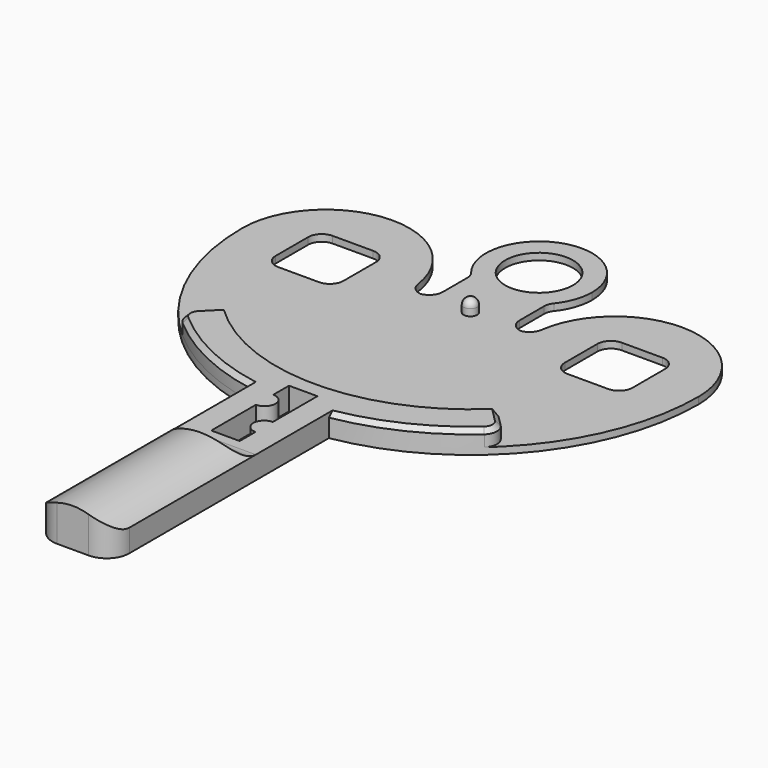
from build123d import *

# Parameters (mm, degrees)
F1_DEPTH     = 5
F3_DEPTH     = 5.001
F5_DEPTH     = 35
F6_T4_DEPTH  = 17.0072864353
F6_S5_R      = 12
F6_T6_DEPTH  = 11
F6_T7_DEPTH  = 30
F7_R         = 7.5
F8_DEPTH     = 5
F9_R         = 45.5
F10_DEPTH    = 3.5
F12_DEPTH    = 1.5
F14_DEPTH    = 3.5
F18_W        = 15
F18_H        = 15
F19_DEPTH    = 1.5010001
F20_DEPTH    = 5.0010001
F21_R        = 1.5
F22_DEPTH    = 3
F23_T1_DEPTH = 1.5
F23_T3_DEPTH = 11.4776669635
F24_R        = 1.5
F25_SIZE     = 1


# Not quite as in the source:
# - a fillet or chamfer that OpenCascade refuses, or shapes differently, is made with other operations: its cross-section is extruded or revolved along the edge and cut away or added
# - a feature names something its author has since deleted; it is built from what else it names


with BuildPart() as f1:
    # F0 (on Top) → F1 (new body)
    with BuildSketch(Plane.XY):
        Polygon((8.5036432176, -40), (-8.5036432176, -40), (-8.5036432176, -110), (0, -110), (8.5036432176, -110), align=None)
    extrude(amount=F1_DEPTH)

    # F2 (on face) → F3 (cut, through all)
    with BuildSketch(Plane.XY.offset(5)):
        with BuildLine():
            Line((-3.15, -67.75), (3.15, -67.75))
            Line((3.15, -67.75), (3.15, -63.4))
            ThreePointArc((3.15, -63.4), (0.75, -61), (3.15, -58.6))
            Line((3.15, -58.6), (3.15, -46.25))
            Line((3.15, -46.25), (-3.15, -46.25))
            Line((-3.15, -46.25), (-3.15, -50.6))
            ThreePointArc((-3.15, -50.6), (-0.75, -53), (-3.15, -55.4))
            Line((-3.15, -55.4), (-3.15, -67.75))
        make_face()
    extrude(amount=-F3_DEPTH, mode=Mode.SUBTRACT)

    # F4 (on face) → F5 (join)
    with BuildSketch(Plane.XZ.offset(110)):
        with BuildLine():
            ThreePointArc((8.5036432176, 5), (0, 8.5331202898), (-8.5036432176, 5))
            Line((-8.5036432176, 5), (8.5036432176, 5))
        make_face()
    extrude(amount=-F5_DEPTH)

    # F6: fillet of radius 5 on 3 edges, made by hand


with BuildPart() as f6_tool2:
    # F6_s3 → F6_t4 (new body)
    with BuildSketch(Plane.YZ.offset(-8.5036432176)):
        with BuildLine():
            ThreePointArc((-70, 5), (-73.5355339059, 6.4644660941), (-75, 10))
            Line((-75, 10), (-75, 5))
            Line((-75, 5), (-70, 5))
        make_face()
    extrude(amount=F6_T4_DEPTH)

    # F6_s5 → F6_t6 (intersect, symmetric)
    with BuildSketch(Plane.XZ.offset(72.5)):
        with Locations((0, -3.4668797102)):
            Circle(F6_S5_R)
    extrude(amount=F6_T6_DEPTH, both=True, mode=Mode.INTERSECT)


with BuildPart() as f1_1:
    add(f1.part)

    # F6_t1: union F6_tool2
    add(f6_tool2.part)

    # F6_s8 → F6_t7 (cut)
    with BuildSketch(Plane.XY.offset(-12.5)):
        with BuildLine():
            ThreePointArc((-8.5036432176, -105), (-7.0391771236, -108.5355339059), (-3.5036432176, -110))
            Line((-3.5036432176, -110), (-8.5036432176, -110))
            Line((-8.5036432176, -110), (-8.5036432176, -105))
        make_face()
        with BuildLine():
            ThreePointArc((8.5036432176, -105), (7.0391771236, -108.5355339059), (3.5036432176, -110))
            Line((3.5036432176, -110), (8.5036432176, -110))
            Line((8.5036432176, -110), (8.5036432176, -105))
        make_face()
    extrude(amount=F6_T7_DEPTH, mode=Mode.SUBTRACT)

    # F7 (on Top) → F8 (join)
    with BuildSketch(Plane.XY):
        with BuildLine():
            Line((-8.5036432176, 0), (-8.5036432176, -40))
            Line((-8.5036432176, -40), (8.5036432176, -40))
            Line((8.5036432176, -40), (8.5036432176, 0))
            Line((8.5036432176, 0), (8.5036432176, 10.8923699759))
            ThreePointArc((8.5036432176, 10.8923699759), (0, 7.2507186355), (-8.5036432176, 10.8923699759))
            Line((-8.5036432176, 10.8923699759), (-8.5036432176, 0))
        make_face()
        with BuildLine():
            ThreePointArc((11.7492813645, 19), (-4.3665727862, 29.9077337098), (-8.5036432176, 10.8923699759))
            ThreePointArc((-8.5036432176, 10.8923699759), (0, 7.2507186355), (8.5036432176, 10.8923699759))
            ThreePointArc((8.5036432176, 10.8923699759), (10.9077337098, 14.6334272138), (11.7492813645, 19))
        make_face()
        with Locations((0, 19)):
            Circle(F7_R, mode=Mode.SUBTRACT)
    extrude(amount=F8_DEPTH)

    # F9 (on face) → F10 (cut)
    with BuildSketch(Plane.XY.offset(5)):
        Circle(F9_R)
    extrude(amount=-F10_DEPTH, mode=Mode.SUBTRACT)

    # F11 (on Top) → F12 (join)
    with BuildSketch(Plane.XY):
        with BuildLine():
            ThreePointArc((-13.5, 0), (-32, 18.5), (-50.5, 0))
            ThreePointArc((-50.5, 0), (0, -50.5), (50.5, 0))
            ThreePointArc((50.5, 0), (32, 18.5), (13.5, 0))
            Line((13.5, 0), (-13.5, 0))
        make_face()
    extrude(amount=F12_DEPTH)

    # F13 (on face) → F14 (join)
    with BuildSketch(Plane.XY.offset(1.5)):
        with BuildLine():
            ThreePointArc((32.173358544, -32.173358544), (0, -45.5), (-32.173358544, -32.173358544))
            Line((-32.173358544, -32.173358544), (-35.7088924499, -35.7088924499))
            ThreePointArc((-35.7088924499, -35.7088924499), (0, -50.5), (35.7088924499, -35.7088924499))
            Line((35.7088924499, -35.7088924499), (32.173358544, -32.173358544))
        make_face()
    extrude(amount=F14_DEPTH)

    # F17: sweep along a path in F17_path
    with BuildLine(Plane(origin=(32.173358544, -32.173358544, 5), x_dir=(0, 1, 0), z_dir=(0, 0, 1))) as f17_path:
        ThreePointArc((0, 0), (-13.326641456, 32.173358544), (0, 64.346717088))
    # F16 (on face) → F17 (sweep)
    with BuildSketch(Plane(origin=(0, 0, 0), x_dir=(0.7071067812, 0.7071067812, 0), z_dir=(0.7071067812, -0.7071067812, 0))):
        Polygon((-43, 5), (-45.5, 5), (-45.5, 2.5), align=None)
    sweep(path=f17_path.line)

    # F18 (on face) → F19 (cut, through all)
    with BuildSketch(Plane.XY.offset(1.5)):
        with Locations((-32, 0)):
            Rectangle(F18_W, F18_H)
        with Locations((32, 0)):
            Rectangle(F18_W, F18_H)
    extrude(amount=-F19_DEPTH, mode=Mode.SUBTRACT)

    # F2 (on face) → F20 (cut, through all)
    with BuildSketch(Plane.XY.offset(5)):
        with BuildLine():
            Line((-3.15, -67.75), (3.15, -67.75))
            Line((3.15, -67.75), (3.15, -63.4))
            ThreePointArc((3.15, -63.4), (0.75, -61), (3.15, -58.6))
            Line((3.15, -58.6), (3.15, -46.25))
            Line((3.15, -46.25), (-3.15, -46.25))
            Line((-3.15, -46.25), (-3.15, -50.6))
            ThreePointArc((-3.15, -50.6), (-0.75, -53), (-3.15, -55.4))
            Line((-3.15, -55.4), (-3.15, -67.75))
        make_face()
    extrude(amount=-F20_DEPTH, mode=Mode.SUBTRACT)

    # F21 (on face) → F22 (join)
    with BuildSketch(Plane.XY.offset(1.5)):
        Circle(F21_R)
    extrude(amount=F22_DEPTH)

    # F23: fillet of radius 3 on 16 edges, made by hand

    # F23_s2 → F23_t1 (join)
    with BuildSketch(Plane.XY):
        with BuildLine():
            ThreePointArc((-10.710331144, 0), (-12.6780946011, 0.7355117627), (-13.6809826122, 2.5813953488))
            ThreePointArc((-13.6809826122, 2.5813953488), (-13.5453011177, 1.2938659758), (-13.5, 0))
            Line((-13.5, 0), (-10.710331144, 0))
        make_face()
        with BuildLine():
            ThreePointArc((13.6809826122, 2.5813953488), (12.6780946011, 0.7355117627), (10.710331144, 0))
            Line((10.710331144, 0), (13.5, 0))
            ThreePointArc((13.5, 0), (13.5453011177, 1.2938659758), (13.6809826122, 2.5813953488))
        make_face()
        with BuildLine():
            ThreePointArc((39.5, -4.5), (38.6213203436, -6.6213203436), (36.5, -7.5))
            Line((36.5, -7.5), (39.5, -7.5))
            Line((39.5, -7.5), (39.5, -4.5))
        make_face()
        with BuildLine():
            ThreePointArc((24.5, -4.5), (25.3786796564, -6.6213203436), (27.5, -7.5))
            Line((27.5, -7.5), (24.5, -7.5))
            Line((24.5, -7.5), (24.5, -4.5))
        make_face()
        with BuildLine():
            ThreePointArc((24.5, 4.5), (25.3786796564, 6.6213203436), (27.5, 7.5))
            Line((27.5, 7.5), (24.5, 7.5))
            Line((24.5, 7.5), (24.5, 4.5))
        make_face()
        with BuildLine():
            ThreePointArc((36.5, 7.5), (38.6213203436, 6.6213203436), (39.5, 4.5))
            Line((39.5, 4.5), (39.5, 7.5))
            Line((39.5, 7.5), (36.5, 7.5))
        make_face()
        with BuildLine():
            ThreePointArc((-27.5, 7.5), (-25.3786796564, 6.6213203436), (-24.5, 4.5))
            Line((-24.5, 4.5), (-24.5, 7.5))
            Line((-24.5, 7.5), (-27.5, 7.5))
        make_face()
        with BuildLine():
            ThreePointArc((-36.5, -7.5), (-38.6213203436, -6.6213203436), (-39.5, -4.5))
            Line((-39.5, -4.5), (-39.5, -7.5))
            Line((-39.5, -7.5), (-36.5, -7.5))
        make_face()
        with BuildLine():
            ThreePointArc((-27.5, -7.5), (-25.3786796564, -6.6213203436), (-24.5, -4.5))
            Line((-24.5, -4.5), (-24.5, -7.5))
            Line((-24.5, -7.5), (-27.5, -7.5))
        make_face()
        with BuildLine():
            ThreePointArc((-39.5, 4.5), (-38.6213203436, 6.6213203436), (-36.5, 7.5))
            Line((-36.5, 7.5), (-39.5, 7.5))
            Line((-39.5, 7.5), (-39.5, 4.5))
        make_face()
        with BuildLine():
            ThreePointArc((11.5036432176, 0), (9.3823228741, 0.8786796564), (8.5036432176, 3))
            Line((8.5036432176, 3), (8.5036432176, 0))
            Line((8.5036432176, 0), (11.5036432176, 0))
        make_face()
        with BuildLine():
            ThreePointArc((-8.5036432176, 3), (-9.3823228741, 0.8786796564), (-11.5036432176, 0))
            Line((-11.5036432176, 0), (-8.5036432176, 0))
            Line((-8.5036432176, 0), (-8.5036432176, 3))
        make_face()
        with BuildLine():
            ThreePointArc((-9.163805174, 11.6467498809), (-8.6734917967, 10.7643189961), (-8.5036432176, 9.7692094873))
            Line((-8.5036432176, 9.7692094873), (-8.5036432176, 10.8923699759))
            ThreePointArc((-8.5036432176, 10.8923699759), (-8.8417733192, 11.2625160968), (-9.163805174, 11.6467498809))
        make_face()
        with BuildLine():
            ThreePointArc((8.5036432176, 9.7692094873), (8.6734917967, 10.7643189961), (9.163805174, 11.6467498809))
            ThreePointArc((9.163805174, 11.6467498809), (8.8417733192, 11.2625160968), (8.5036432176, 10.8923699759))
            Line((8.5036432176, 10.8923699759), (8.5036432176, 9.7692094873))
        make_face()
    extrude(amount=F23_T1_DEPTH)

    # F23_s4 → F23_t3 (cut)
    with BuildSketch(Plane.XY.offset(1.5)):
        with BuildLine():
            ThreePointArc((33.382302863, -37.8928998041), (34.3976980488, -35.7366206113), (33.5205161058, -33.5205161058))
            Line((33.5205161058, -33.5205161058), (35.7088924499, -35.7088924499))
            ThreePointArc((35.7088924499, -35.7088924499), (34.5628527392, -36.8192777024), (33.382302863, -37.8928998041))
        make_face()
        with BuildLine():
            ThreePointArc((-33.382302863, -37.8928998041), (-34.3976980488, -35.7366206113), (-33.5205161058, -33.5205161058))
            Line((-33.5205161058, -33.5205161058), (-35.7088924499, -35.7088924499))
            ThreePointArc((-35.7088924499, -35.7088924499), (-34.5628527392, -36.8192777024), (-33.382302863, -37.8928998041))
        make_face()
    extrude(amount=F23_T3_DEPTH, mode=Mode.SUBTRACT)

    # F24
    f24_edges = [f1_1.edges().sort_by_distance(p)[0] for p in [
        (-1.5, 0, 4.5),
    ]]
    fillet(f24_edges, radius=F24_R)

    # F25
    f25_edges = [f1_1.edges().sort_by_distance(p)[0] for p in [
        (21.769872, -45.566684, 5),
        (-21.769872, -45.566684, 5),
        (-34.397698, -35.736621, 5),
        (-31.963054, -31.963054, 5),
        (31.963054, -31.963054, 5),
        (34.397698, -35.736621, 5),
    ]]
    chamfer(f25_edges, length=F25_SIZE)


solid = f1_1.part
